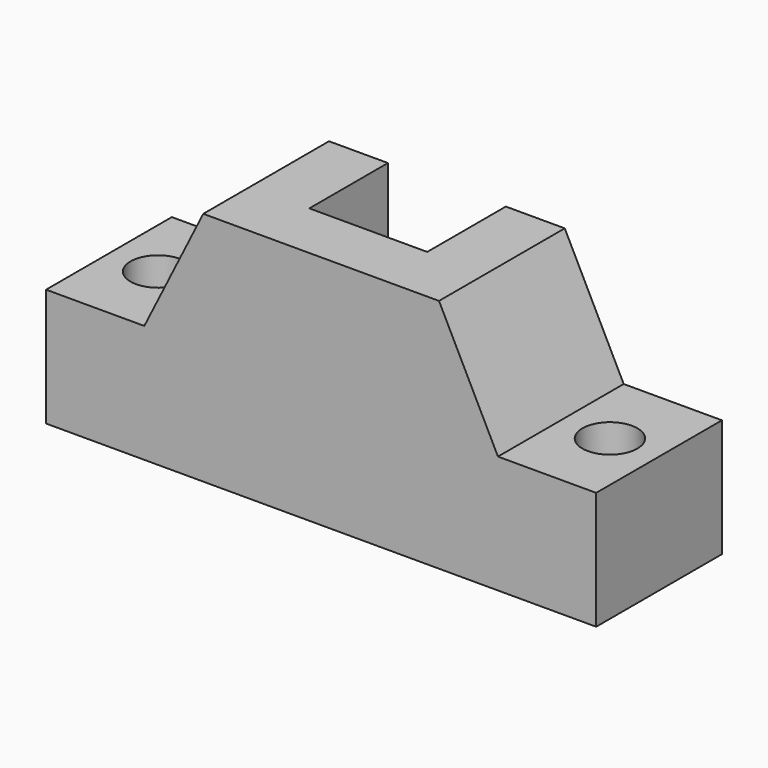
from build123d import *

# Parameters (mm, degrees)
F1_DEPTH      = 40
F2_SIZE2      = 14.99999
F2_SIZE       = 29.99999
F2_2_SIZE2    = 14.99999
F2_2_SIZE     = 29.99999
F3_W          = 30
F3_H          = 45
F4_DEPTH      = 25
F5_SIZE2      = 24.99999
F5_SIZE       = 44.99999
F6_R          = 7
F7_DEPTH      = 15
F7_DEPTH_BACK = 20


# Not quite as in the source:
# - a fillet or chamfer is up to 0.001 mm smaller than in the source, because OpenCascade refuses the exact size


with BuildPart() as f1:
    # F0 (on Front) → F1 (new body)
    with BuildSketch(Plane.XZ):
        Polygon((20.7067526877, 42.941089198), (-69.2932473123, 42.941089198), (-69.2932473123, 12.941089198), (-94.2932473123, 12.941089198), (-94.2932473123, -17.058910802), (45.7067526877, -17.058910802), (45.7067526877, 12.941089198), (20.7067526877, 12.941089198), align=None)
    extrude(amount=F1_DEPTH)

    # F2 (size 30 and 15 in the source; OpenCascade refuses exactly that, so slightly less here)
    f2_edges = [f1.edges().sort_by_distance(p)[0] for p in [
        (-69.293247, -20, 42.941089),
    ]]
    f2_side = f1.faces().sort_by_distance((-69.293247, -20, 27.941089))[0]
    chamfer(f2_edges, length=F2_SIZE, length2=F2_SIZE2, reference=f2_side)

    # F2#2 (size 30 and 15 in the source; OpenCascade refuses exactly that, so slightly less here)
    f2_2_edges = [f1.edges().sort_by_distance(p)[0] for p in [
        (20.706753, -20, 42.941089),
    ]]
    f2_2_side = f1.faces().sort_by_distance((20.706753, -20, 27.941089))[0]
    chamfer(f2_2_edges, length=F2_2_SIZE, length2=F2_2_SIZE2, reference=f2_2_side)

    # F3 (on Front) → F4 (cut)
    with BuildSketch(Plane.XZ):
        with Locations((-24.2932473123, 20.441089198)):
            Rectangle(F3_W, F3_H)
    extrude(amount=F4_DEPTH, mode=Mode.SUBTRACT)

    # F5 (size 45 and 25 in the source; OpenCascade refuses exactly that, so slightly less here)
    f5_edges = [f1.edges().sort_by_distance(p)[0] for p in [
        (-24.293247, -25, -2.058911),
    ]]
    f5_side = f1.faces().sort_by_distance((-24.293247, -25, 20.441089))[0]
    chamfer(f5_edges, length=F5_SIZE, length2=F5_SIZE2, reference=f5_side)

    # F6 (on Top) → F7 (cut, two sides)
    with BuildSketch(Plane.XY) as f7_sk:
        with Locations((-81.7932473123, -20)):
            Circle(F6_R)
        with Locations((33.2067526877, -20)):
            Circle(F6_R)
    extrude(amount=F7_DEPTH, mode=Mode.SUBTRACT)
    extrude(f7_sk.sketch, amount=-F7_DEPTH_BACK, mode=Mode.SUBTRACT)


solid = f1.part
